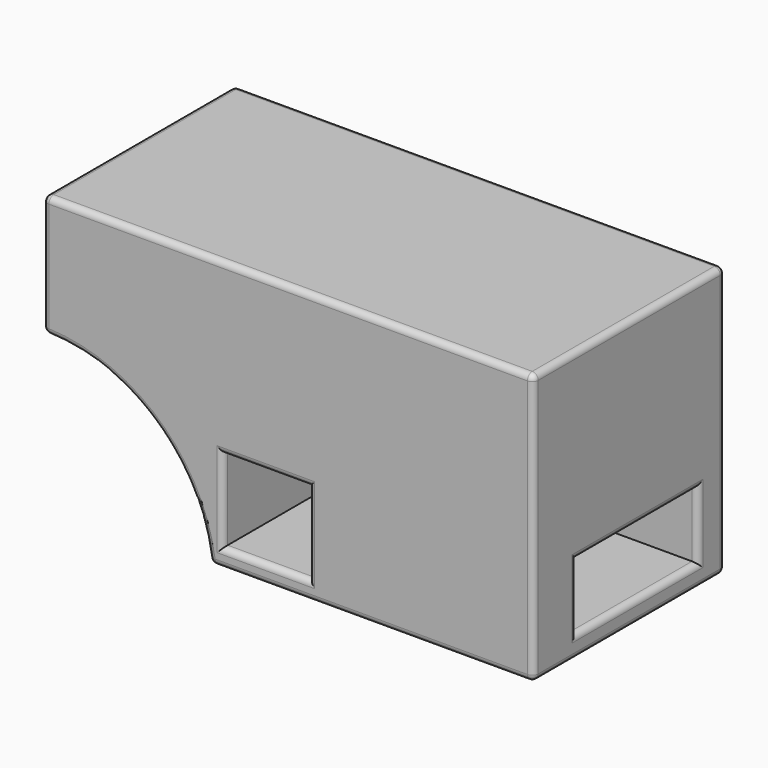
from build123d import *

# Parameters (mm, degrees)
F0_W         = 9.105252102
F0_H         = 8.7177967653
F1_DEPTH     = 25.4
F2_W         = 16.0794917028
F2_H         = 6.9742375053
F3_DEPTH     = 23.8286424428
F4_R         = 0.635
F5_T1_DEPTH  = 16.0794917028
F5_T3_DEPTH  = 6.9742375053
F5_T5_DEPTH  = 8.7177967653
F5_T7_DEPTH  = 9.105252102
F5_T13_DEPTH = 17.6669917028
F5_T17_DEPTH = 8.5617375053
F5_T25_DEPTH = 17.6669917028
F5_T29_DEPTH = 8.5617375053
F5_T37_DEPTH = 8.5617375053
F5_T42_DEPTH = 17.5413992589
F5_T49_DEPTH = 17.5413992589
F5_T53_DEPTH = 8.5617375053
F5_T61_DEPTH = 10.3052967653
F5_T65_DEPTH = 10.692752102
F5_T72_DEPTH = 10.692752102
F5_T76_DEPTH = 10.3052967653
F5_T83_DEPTH = 10.692752102
F5_T87_DEPTH = 10.3052967653
F5_T94_DEPTH = 10.3052967653
F5_T98_DEPTH = 10.692752102
F6_R         = 0.635


# Not quite as in the source:
# - a fillet or chamfer that OpenCascade refuses, or shapes differently, is made with other operations: its cross-section is extruded or revolved along the edge and cut away or added


with BuildPart() as f1:
    # F0 (on Front) → F1 (new body)
    with BuildSketch(Plane.XZ):
        with BuildLine():
            ThreePointArc((0, 17.8214723471), (11.860718486, 13.3014372763), (17.7050021368, 2.0341523923))
            Line((17.7050021368, 2.0341523923), (52.0161837339, 2.0341523923))
            Line((52.0161837339, 2.0341523923), (52.0161837339, 30.7060163468))
            Line((52.0161837339, 30.7060163468), (0, 30.7060163468))
            Line((0, 30.7060163468), (0, 17.8214723471))
        make_face()
        with Locations((23.6349152401, 8.3303391002)):
            Rectangle(F0_W, F0_H, mode=Mode.SUBTRACT)
    extrude(amount=F1_DEPTH)

    # F2 (on face) → F3 (cut, through all)
    with BuildSketch(Plane.YZ.offset(52.0161837339)):
        with Locations((-11.6237296024, 7.8460171353)):
            Rectangle(F2_W, F2_H)
    extrude(amount=-F3_DEPTH, mode=Mode.SUBTRACT)

    # F4
    f4_edges = [f1.edges().sort_by_distance(p)[0] for p in [
        (23.634915, -25.4, 3.971441),
        (19.082289, -25.4, 8.330339),
        (23.634915, -25.4, 12.689237),
        (28.187541, -25.4, 8.330339),
        (52.016184, -11.62373, 4.358898),
        (52.016184, -19.663475, 7.846017),
        (52.016184, -11.62373, 11.333136),
        (52.016184, -3.583984, 7.846017),
    ]]
    fillet(f4_edges, radius=F4_R)

    # F5: fillet of radius 0.635 on 8 edges, made by hand

    # F5_s2 → F5_t1 (cut)
    with BuildSketch(Plane.XZ.offset(3.583983751)):
        with BuildLine():
            ThreePointArc((28.1875412911, 11.968135888), (28.3735284851, 11.5191230819), (28.8225412911, 11.333135888))
            Line((28.8225412911, 11.333135888), (28.1875412911, 11.333135888))
            Line((28.1875412911, 11.333135888), (28.1875412911, 11.968135888))
        make_face()
        with BuildLine():
            ThreePointArc((28.1875412911, 3.9714407176), (28.421565367, 4.2532443861), (28.7723043136, 4.3588983826))
            Line((28.7723043136, 4.3588983826), (28.1875412911, 4.3588983826))
            Line((28.1875412911, 4.3588983826), (28.1875412911, 3.9714407176))
        make_face()
    extrude(amount=F5_T1_DEPTH, mode=Mode.SUBTRACT)

    # F5_s4 → F5_t3 (cut)
    with BuildSketch(Plane.XY.offset(4.3588983826)):
        with BuildLine():
            ThreePointArc((28.1875412911, -20.2984754539), (28.3735284851, -19.8494626478), (28.8225412911, -19.6634754539))
            Line((28.8225412911, -19.6634754539), (28.1875412911, -19.6634754539))
            Line((28.1875412911, -19.6634754539), (28.1875412911, -20.2984754539))
        make_face()
        with BuildLine():
            ThreePointArc((28.1875412911, -2.948983751), (28.3735284851, -3.3979965571), (28.8225412911, -3.583983751))
            Line((28.8225412911, -3.583983751), (28.1875412911, -3.583983751))
            Line((28.1875412911, -3.583983751), (28.1875412911, -2.948983751))
        make_face()
    extrude(amount=F5_T3_DEPTH, mode=Mode.SUBTRACT)

    # F5_s6 → F5_t5 (cut)
    with BuildSketch(Plane.XY.offset(3.9714407176)):
        with BuildLine():
            ThreePointArc((28.1875412911, -0.635), (28.3735284851, -0.1859871939), (28.8225412911, 0))
            Line((28.8225412911, 0), (28.1875412911, 0))
            Line((28.1875412911, 0), (28.1875412911, -0.635))
        make_face()
        with BuildLine():
            ThreePointArc((19.0822891891, -0.635), (18.8963019952, -0.1859871939), (18.4472891891, 0))
            Line((18.4472891891, 0), (19.0822891891, 0))
            Line((19.0822891891, 0), (19.0822891891, -0.635))
        make_face()
    extrude(amount=F5_T5_DEPTH, mode=Mode.SUBTRACT)

    # F5_s8 → F5_t7 (cut)
    with BuildSketch(Plane.YZ.offset(19.0822891891)):
        with BuildLine():
            ThreePointArc((-0.635, 12.6892374828), (-0.1859871939, 12.8752246768), (0, 13.3242374828))
            Line((0, 13.3242374828), (0, 12.6892374828))
            Line((0, 12.6892374828), (-0.635, 12.6892374828))
        make_face()
        with BuildLine():
            ThreePointArc((-0.635, 3.9714407176), (-0.1859871939, 3.7854535236), (0, 3.3364407176))
            Line((0, 3.3364407176), (0, 3.9714407176))
            Line((0, 3.9714407176), (-0.635, 3.9714407176))
        make_face()
    extrude(amount=F5_T7_DEPTH, mode=Mode.SUBTRACT)


with BuildPart() as f5_tool11:
    # F5_s12 → F5_t13 (new body)
    with BuildSketch(Plane.XZ.offset(1.996483751)):
        with BuildLine():
            ThreePointArc((28.1875412911, 11.968135888), (28.3735284851, 11.5191230819), (28.8225412911, 11.333135888))
            Line((28.8225412911, 11.333135888), (28.1875412911, 11.333135888))
            Line((28.1875412911, 11.333135888), (28.1875412911, 11.968135888))
        make_face()
    extrude(amount=F5_T13_DEPTH)

    split(bisect_by=Plane.XZ.offset(3.583983751), keep=Keep.BOTTOM)


with BuildPart() as f5_tool15:
    # F5_s16 → F5_t17 (new body)
    with BuildSketch(Plane.XY.offset(4.3588983826)):
        with BuildLine():
            ThreePointArc((28.1875412911, -2.948983751), (28.3735284851, -3.3979965571), (28.8225412911, -3.583983751))
            Line((28.8225412911, -3.583983751), (28.1875412911, -3.583983751))
            Line((28.1875412911, -3.583983751), (28.1875412911, -2.948983751))
        make_face()
    extrude(amount=F5_T17_DEPTH)

    split(bisect_by=Plane.XY.offset(12.6892374828), keep=Keep.BOTTOM)

    split(bisect_by=Plane.XY.offset(11.333135888), keep=Keep.TOP)


with BuildPart() as f5_tool11_1:
    add(f5_tool11.part)

    # F5_t20: intersect F5_tool15
    add(f5_tool15.part, mode=Mode.INTERSECT)


with BuildPart() as f1_1:
    add(f1.part)

    # F5_t9: cut F5_tool11
    add(f5_tool11_1.part, mode=Mode.SUBTRACT)


with BuildPart() as f5_tool23:
    # F5_s24 → F5_t25 (new body)
    with BuildSketch(Plane.XZ.offset(3.583983751)):
        with BuildLine():
            ThreePointArc((28.1875412911, 11.968135888), (28.3735284851, 11.5191230819), (28.8225412911, 11.333135888))
            Line((28.8225412911, 11.333135888), (28.1875412911, 11.333135888))
            Line((28.1875412911, 11.333135888), (28.1875412911, 11.968135888))
        make_face()
    extrude(amount=F5_T25_DEPTH)

    split(bisect_by=Plane.XZ.offset(19.6634754539), keep=Keep.TOP)


with BuildPart() as f5_tool27:
    # F5_s28 → F5_t29 (new body)
    with BuildSketch(Plane.XY.offset(12.920635888)):
        with BuildLine():
            ThreePointArc((28.1875412911, -20.2984754539), (28.3735284851, -19.8494626478), (28.8225412911, -19.6634754539))
            Line((28.8225412911, -19.6634754539), (28.1875412911, -19.6634754539))
            Line((28.1875412911, -19.6634754539), (28.1875412911, -20.2984754539))
        make_face()
    extrude(amount=-F5_T29_DEPTH)

    split(bisect_by=Plane.XY.offset(12.6892374828), keep=Keep.BOTTOM)

    split(bisect_by=Plane.XY.offset(11.333135888), keep=Keep.TOP)


with BuildPart() as f5_tool23_1:
    add(f5_tool23.part)

    # F5_t32: intersect F5_tool27
    add(f5_tool27.part, mode=Mode.INTERSECT)


with BuildPart() as f1_2:
    add(f1_1.part)

    # F5_t21: cut F5_tool23
    add(f5_tool23_1.part, mode=Mode.SUBTRACT)


with BuildPart() as f5_tool35:
    # F5_s36 → F5_t37 (new body)
    with BuildSketch(Plane.XY.offset(11.333135888)):
        with BuildLine():
            ThreePointArc((28.1875412911, -20.2984754539), (28.3735284851, -19.8494626478), (28.8225412911, -19.6634754539))
            Line((28.8225412911, -19.6634754539), (28.1875412911, -19.6634754539))
            Line((28.1875412911, -19.6634754539), (28.1875412911, -20.2984754539))
        make_face()
    extrude(amount=-F5_T37_DEPTH)

    split(bisect_by=Plane.XY.offset(3.9714407176), keep=Keep.TOP)

    split(bisect_by=Plane.XY.offset(4.3588983826), keep=Keep.BOTTOM)


with BuildPart() as f5_tool40:
    # F5_s41 → F5_t42 (new body)
    with BuildSketch(Plane.XZ.offset(21.1253830099)):
        with BuildLine():
            ThreePointArc((28.1875412911, 3.9714407176), (28.421565367, 4.2532443861), (28.7723043136, 4.3588983826))
            Line((28.7723043136, 4.3588983826), (28.1875412911, 4.3588983826))
            Line((28.1875412911, 4.3588983826), (28.1875412911, 3.9714407176))
        make_face()
    extrude(amount=-F5_T42_DEPTH)

    split(bisect_by=Plane.XZ.offset(19.6634754539), keep=Keep.TOP)


with BuildPart() as f5_tool35_1:
    add(f5_tool35.part)

    # F5_t44: intersect F5_tool40
    add(f5_tool40.part, mode=Mode.INTERSECT)


with BuildPart() as f1_3:
    add(f1_2.part)

    # F5_t33: cut F5_tool35
    add(f5_tool35_1.part, mode=Mode.SUBTRACT)


with BuildPart() as f5_tool47:
    # F5_s48 → F5_t49 (new body)
    with BuildSketch(Plane.XZ.offset(19.6634754539)):
        with BuildLine():
            ThreePointArc((28.1875412911, 3.9714407176), (28.421565367, 4.2532443861), (28.7723043136, 4.3588983826))
            Line((28.7723043136, 4.3588983826), (28.1875412911, 4.3588983826))
            Line((28.1875412911, 4.3588983826), (28.1875412911, 3.9714407176))
        make_face()
    extrude(amount=-F5_T49_DEPTH)

    split(bisect_by=Plane.XZ.offset(3.583983751), keep=Keep.BOTTOM)


with BuildPart() as f5_tool51:
    # F5_s52 → F5_t53 (new body)
    with BuildSketch(Plane.XY.offset(2.7713983826)):
        with BuildLine():
            ThreePointArc((28.1875412911, -2.948983751), (28.3735284851, -3.3979965571), (28.8225412911, -3.583983751))
            Line((28.8225412911, -3.583983751), (28.1875412911, -3.583983751))
            Line((28.1875412911, -3.583983751), (28.1875412911, -2.948983751))
        make_face()
    extrude(amount=F5_T53_DEPTH)

    split(bisect_by=Plane.XY.offset(3.9714407176), keep=Keep.TOP)

    split(bisect_by=Plane.XY.offset(4.3588983826), keep=Keep.BOTTOM)


with BuildPart() as f5_tool47_1:
    add(f5_tool47.part)

    # F5_t56: intersect F5_tool51
    add(f5_tool51.part, mode=Mode.INTERSECT)


with BuildPart() as f1_4:
    add(f1_3.part)

    # F5_t45: cut F5_tool47
    add(f5_tool47_1.part, mode=Mode.SUBTRACT)


with BuildPart() as f5_tool59:
    # F5_s60 → F5_t61 (new body)
    with BuildSketch(Plane.XY.offset(14.2767374828)):
        with BuildLine():
            ThreePointArc((28.1875412911, -0.635), (28.3735284851, -0.1859871939), (28.8225412911, 0))
            Line((28.8225412911, 0), (28.1875412911, 0))
            Line((28.1875412911, 0), (28.1875412911, -0.635))
        make_face()
    extrude(amount=-F5_T61_DEPTH)

    split(bisect_by=Plane.XY.offset(12.6892374828), keep=Keep.TOP)


with BuildPart() as f5_tool63:
    # F5_s64 → F5_t65 (new body)
    with BuildSketch(Plane.YZ.offset(19.0822891891)):
        with BuildLine():
            ThreePointArc((-0.635, 12.6892374828), (-0.1859871939, 12.8752246768), (0, 13.3242374828))
            Line((0, 13.3242374828), (0, 12.6892374828))
            Line((0, 12.6892374828), (-0.635, 12.6892374828))
        make_face()
    extrude(amount=F5_T65_DEPTH)

    split(bisect_by=Plane.YZ.offset(28.1875412911), keep=Keep.TOP)


with BuildPart() as f5_tool59_1:
    add(f5_tool59.part)

    # F5_t67: intersect F5_tool63
    add(f5_tool63.part, mode=Mode.INTERSECT)


with BuildPart() as f1_5:
    add(f1_4.part)

    # F5_t57: cut F5_tool59
    add(f5_tool59_1.part, mode=Mode.SUBTRACT)


with BuildPart() as f5_tool70:
    # F5_s71 → F5_t72 (new body)
    with BuildSketch(Plane.YZ.offset(29.7750412911)):
        with BuildLine():
            ThreePointArc((-0.635, 3.9714407176), (-0.1859871939, 3.7854535236), (0, 3.3364407176))
            Line((0, 3.3364407176), (0, 3.9714407176))
            Line((0, 3.9714407176), (-0.635, 3.9714407176))
        make_face()
    extrude(amount=-F5_T72_DEPTH)

    split(bisect_by=Plane.YZ.offset(28.1875412911), keep=Keep.TOP)


with BuildPart() as f5_tool74:
    # F5_s75 → F5_t76 (new body)
    with BuildSketch(Plane.XY.offset(12.6892374828)):
        with BuildLine():
            ThreePointArc((28.1875412911, -0.635), (28.3735284851, -0.1859871939), (28.8225412911, 0))
            Line((28.8225412911, 0), (28.1875412911, 0))
            Line((28.1875412911, 0), (28.1875412911, -0.635))
        make_face()
    extrude(amount=-F5_T76_DEPTH)

    split(bisect_by=Plane.XY.offset(3.9714407176), keep=Keep.BOTTOM)


with BuildPart() as f5_tool70_1:
    add(f5_tool70.part)

    # F5_t78: intersect F5_tool74
    add(f5_tool74.part, mode=Mode.INTERSECT)


with BuildPart() as f1_6:
    add(f1_5.part)

    # F5_t68: cut F5_tool70
    add(f5_tool70_1.part, mode=Mode.SUBTRACT)


with BuildPart() as f5_tool81:
    # F5_s82 → F5_t83 (new body)
    with BuildSketch(Plane.YZ.offset(28.1875412911)):
        with BuildLine():
            ThreePointArc((-0.635, 3.9714407176), (-0.1859871939, 3.7854535236), (0, 3.3364407176))
            Line((0, 3.3364407176), (0, 3.9714407176))
            Line((0, 3.9714407176), (-0.635, 3.9714407176))
        make_face()
    extrude(amount=-F5_T83_DEPTH)

    split(bisect_by=Plane.YZ.offset(19.0822891891), keep=Keep.BOTTOM)


with BuildPart() as f5_tool85:
    # F5_s86 → F5_t87 (new body)
    with BuildSketch(Plane.XY.offset(2.3839407176)):
        with BuildLine():
            ThreePointArc((19.0822891891, -0.635), (18.8963019952, -0.1859871939), (18.4472891891, 0))
            Line((18.4472891891, 0), (19.0822891891, 0))
            Line((19.0822891891, 0), (19.0822891891, -0.635))
        make_face()
    extrude(amount=F5_T87_DEPTH)

    split(bisect_by=Plane.XY.offset(3.9714407176), keep=Keep.BOTTOM)


with BuildPart() as f5_tool81_1:
    add(f5_tool81.part)

    # F5_t89: intersect F5_tool85
    add(f5_tool85.part, mode=Mode.INTERSECT)


with BuildPart() as f1_7:
    add(f1_6.part)

    # F5_t79: cut F5_tool81
    add(f5_tool81_1.part, mode=Mode.SUBTRACT)


with BuildPart() as f5_tool92:
    # F5_s93 → F5_t94 (new body)
    with BuildSketch(Plane.XY.offset(3.9714407176)):
        with BuildLine():
            ThreePointArc((19.0822891891, -0.635), (18.8963019952, -0.1859871939), (18.4472891891, 0))
            Line((18.4472891891, 0), (19.0822891891, 0))
            Line((19.0822891891, 0), (19.0822891891, -0.635))
        make_face()
    extrude(amount=F5_T94_DEPTH)

    split(bisect_by=Plane.XY.offset(12.6892374828), keep=Keep.TOP)


with BuildPart() as f5_tool96:
    # F5_s97 → F5_t98 (new body)
    with BuildSketch(Plane.YZ.offset(17.4947891891)):
        with BuildLine():
            ThreePointArc((-0.635, 12.6892374828), (-0.1859871939, 12.8752246768), (0, 13.3242374828))
            Line((0, 13.3242374828), (0, 12.6892374828))
            Line((0, 12.6892374828), (-0.635, 12.6892374828))
        make_face()
    extrude(amount=F5_T98_DEPTH)

    split(bisect_by=Plane.YZ.offset(19.0822891891), keep=Keep.BOTTOM)


with BuildPart() as f5_tool92_1:
    add(f5_tool92.part)

    # F5_t100: intersect F5_tool96
    add(f5_tool96.part, mode=Mode.INTERSECT)


with BuildPart() as f1_8:
    add(f1_7.part)

    # F5_t90: cut F5_tool92
    add(f5_tool92_1.part, mode=Mode.SUBTRACT)

    # F6
    f6_edges = [f1_8.edges().sort_by_distance(p)[0] for p in [
        (11.860718, 0, 13.301437),
        (11.860718, -25.4, 13.301437),
        (17.705002, -12.7, 2.034152),
        (0, -12.7, 17.821472),
        (0, 0, 24.263744),
        (0, -25.4, 24.263744),
        (26.008092, 0, 30.706016),
        (52.016184, 0, 16.370084),
        (34.860593, 0, 2.034152),
        (52.016184, -12.7, 30.706016),
        (52.016184, -25.4, 16.370084),
        (52.016184, -12.7, 2.034152),
        (26.008092, -25.4, 30.706016),
        (0, -12.7, 30.706016),
        (34.860593, -25.4, 2.034152),
    ]]
    fillet(f6_edges, radius=F6_R)


solid = f1_8.part
